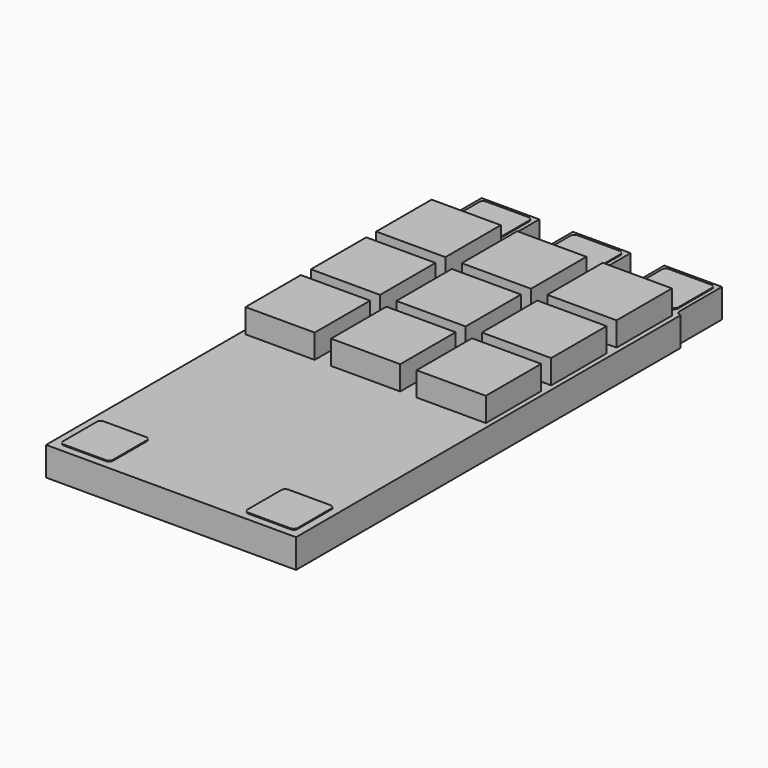
from build123d import *

# Parameters (mm, degrees)
F0_W      = 13
F0_H      = 28
F1_DEPTH  = 1.5
F2_W      = 1.75
F2_H      = 3
F2_W_2    = 0.25
F3_DEPTH  = 25
F4_W      = 2.6
F4_H      = 2.6
F5_DEPTH  = 0.05
F6_R      = 0.2
F7_R      = 0.24999
F8_W      = 2.6
F8_H      = 2.6
F9_DEPTH  = 0.05
F10_R     = 0.2
F11_W     = 3.6
F11_H     = 3.6
F12_DEPTH = 1.25
F13_W     = 7
F13_H     = 7
F14_DEPTH = 1.25


# Not quite as in the source:
# - a fillet or chamfer is up to 0.001 mm smaller than in the source, because OpenCascade refuses the exact size


with BuildPart() as f1:
    # F0 (on Top) → F1 (new body)
    with BuildSketch(Plane.XY):
        Rectangle(F0_W, F0_H)
    extrude(amount=F1_DEPTH)

    # F2 (on face) → F3 (cut)
    with BuildSketch(Plane.XY.offset(1.5)):
        with Locations((-2.375, 12.5)):
            Rectangle(F2_W, F2_H)
        with Locations((2.375, 12.5)):
            Rectangle(F2_W, F2_H)
        with Locations((-6.375, 12.5)):
            Rectangle(F2_W_2, F2_H)
        with Locations((6.375, 12.5)):
            Rectangle(F2_W_2, F2_H)
    extrude(amount=-F3_DEPTH, mode=Mode.SUBTRACT)

    # F4 (on face) → F5 (join)
    with BuildSketch(Plane.XY.offset(1.5)):
        with Locations((-4.75, 12.5)):
            Rectangle(F4_W, F4_H)
        with Locations((0, 12.5)):
            Rectangle(F4_W, F4_H)
        with Locations((4.75, 12.5)):
            Rectangle(F4_W, F4_H)
    extrude(amount=F5_DEPTH)

    # F6
    f6_edges = [f1.edges().sort_by_distance(p)[0] for p in [
        (-6.05, 11.2, 1.525),
        (-6.05, 13.8, 1.525),
        (-3.45, 11.2, 1.525),
        (-3.45, 13.8, 1.525),
        (1.3, 13.8, 1.525),
        (-1.3, 13.8, 1.525),
        (1.3, 11.2, 1.525),
        (3.45, 13.8, 1.525),
        (6.05, 13.8, 1.525),
        (6.05, 11.2, 1.525),
        (-1.3, 11.2, 1.525),
        (3.45, 11.2, 1.525),
    ]]
    fillet(f6_edges, radius=F6_R)

    # F7 (radius 0.25 in the source; OpenCascade refuses exactly that, so slightly less here)
    f7_edges = [f1.edges().sort_by_distance(p)[0] for p in [
        (6.25, 11, 0.75),
        (-6.25, 11, 0.75),
        (-1.5, 11, 0.75),
        (3.25, 11, 0.75),
        (-3.25, 11, 0.75),
        (1.5, 11, 0.75),
    ]]
    fillet(f7_edges, radius=F7_R)

    # F8 (on face) → F9 (join)
    with BuildSketch(Plane.XY.offset(1.5)):
        with Locations((-4.8, -12.3)):
            Rectangle(F8_W, F8_H)
        with Locations((4.8, -12.3)):
            Rectangle(F8_W, F8_H)
    extrude(amount=F9_DEPTH)

    # F10
    f10_edges = [f1.edges().sort_by_distance(p)[0] for p in [
        (-6.1, -13.6, 1.525),
        (-3.5, -13.6, 1.525),
        (-6.1, -11, 1.525),
        (3.5, -13.6, 1.525),
        (6.1, -13.6, 1.525),
        (3.5, -11, 1.525),
        (-3.5, -11, 1.525),
        (6.1, -11, 1.525),
    ]]
    fillet(f10_edges, radius=F10_R)

    # F11 (on face) → F12 (join)
    with BuildSketch(Plane.XY.offset(1.5)):
        with Locations((-4.45, 8.95)):
            Rectangle(F11_W, F11_H)
        with Locations((0, 8.95)):
            Rectangle(F11_W, F11_H)
        with Locations((4.45, 8.95)):
            Rectangle(F11_W, F11_H)
        with Locations((4.45, 4.7)):
            Rectangle(F11_W, F11_H)
        with Locations((0, 4.7)):
            Rectangle(F11_W, F11_H)
        with Locations((-4.45, 4.7)):
            Rectangle(F11_W, F11_H)
        with Locations((4.45, 0.45)):
            Rectangle(F11_W, F11_H)
        with Locations((0, 0.45)):
            Rectangle(F11_W, F11_H)
        with Locations((-4.45, 0.45)):
            Rectangle(F11_W, F11_H)
    extrude(amount=F12_DEPTH)

    # F13 (on face) → F14 (join)
    with BuildSketch(Plane(origin=(0, 0, 0), x_dir=(1, 0, 0), z_dir=(0, 0, -1))):
        with Locations((0, -6)):
            Rectangle(F13_W, F13_H)
        with Locations((0, 6)):
            Rectangle(F13_W, F13_H)
    extrude(amount=F14_DEPTH)


solid = f1.part
